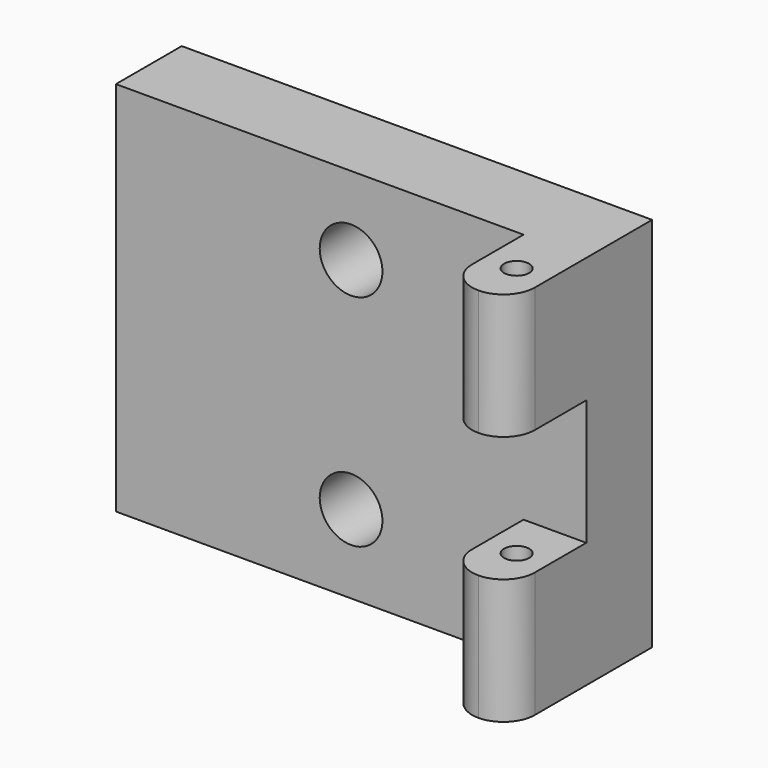
from build123d import *

# Parameters (mm, degrees)
F0_W     = 15
F0_H     = 12
F1_DEPTH = 2.625
F2_W     = 2
F2_H     = 4
F3_DEPTH = 3.05
F4_R     = 0.4
F5_DEPTH = 25
F6_R     = 0.99999
F7_R     = 1
F8_DEPTH = 25


# Not quite as in the source:
# - a fillet or chamfer is up to 0.001 mm smaller than in the source, because OpenCascade refuses the exact size


with BuildPart() as f1:
    # F0 (on Front) → F1 (new body)
    with BuildSketch(Plane.XZ):
        Rectangle(F0_W, F0_H)
    extrude(amount=F1_DEPTH)

    # F2 (on face) → F3 (join)
    with BuildSketch(Plane.XZ.offset(2.625)):
        with Locations((6.5, 4)):
            Rectangle(F2_W, F2_H)
        with Locations((6.5, -4)):
            Rectangle(F2_W, F2_H)
    extrude(amount=F3_DEPTH)

    # F4 (on face) → F5 (cut)
    with BuildSketch(Plane(origin=(0, 0, -6), x_dir=(1, 0, 0), z_dir=(0, 0, -1))):
        with Locations((6.5, 4.15)):
            Circle(F4_R)
    extrude(amount=-F5_DEPTH, mode=Mode.SUBTRACT)

    # F6 (radius 1 in the source; OpenCascade refuses exactly that, so slightly less here)
    f6_edges = [f1.edges().sort_by_distance(p)[0] for p in [
        (7.5, -5.675, 4),
        (5.5, -5.675, 4),
        (7.5, -5.675, -4),
        (5.5, -5.675, -4),
    ]]
    fillet(f6_edges, radius=F6_R)

    # F7 (on face) → F8 (cut)
    with BuildSketch(Plane(origin=(0, 0, 0), x_dir=(-1, 0, 0), z_dir=(0, 1, 0))):
        with Locations((0, 3.5)):
            Circle(F7_R)
        with Locations((0, -3.5)):
            Circle(F7_R)
    extrude(amount=-F8_DEPTH, mode=Mode.SUBTRACT)


solid = f1.part
